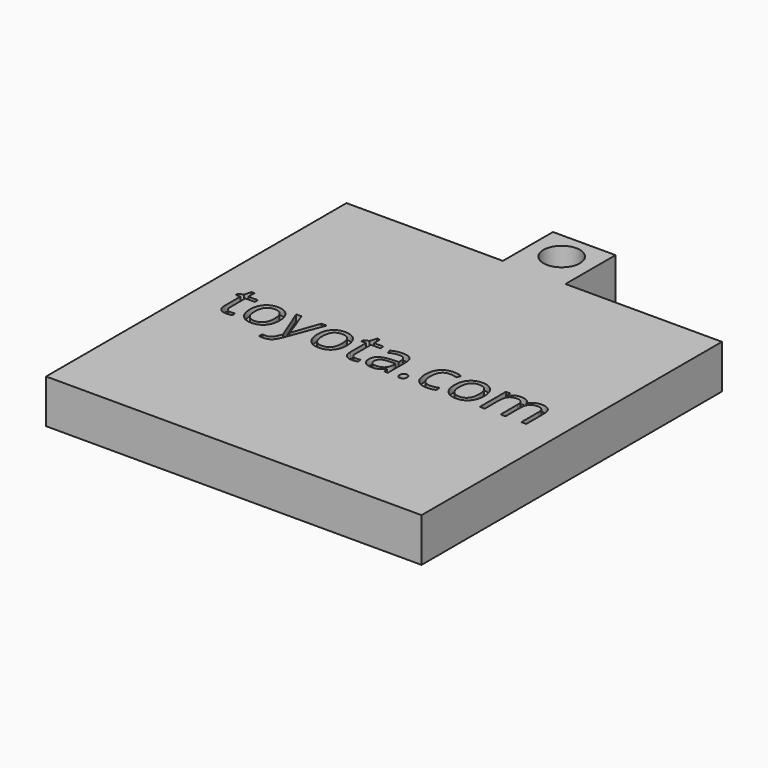
from build123d import *

# Parameters (mm, degrees)
F0_W          = 30
F0_H          = 30
F1_DEPTH      = 1.75
F2_W          = 5
F2_H          = 5
F3_DEPTH      = 3.5
F4_R          = 1.4562657213
F5_DEPTH      = 3.501
F7_DEPTH      = 0.5
F9_DEPTH      = 1.5
F11_DEPTH     = 1.5
F12_TEXT_SIZE = 4.8596224339
F13_DEPTH     = 0.5
F15_DEPTH     = 0.5
F16_W         = 3
F16_H         = 3
F16_W_2       = 2
F16_H_2       = 1
F17_DEPTH     = 0.5


# Not quite as in the source:
# - Text() gives the source's letters only with a copy of the font that has no kerning and outlines rounded to 1/6400 em; it was checked with that copy


with BuildPart() as f1:
    # F0 (on Top) → F1 (new body, symmetric)
    with BuildSketch(Plane.XY):
        Rectangle(F0_W, F0_H)
    extrude(amount=F1_DEPTH, both=True)

    # F2 (on face) → F3 (join)
    with BuildSketch(Plane.XY.offset(1.75)):
        with Locations((0, 17.5)):
            Rectangle(F2_W, F2_H)
    extrude(amount=-F3_DEPTH)

    # F4 (on face) → F5 (cut, through all)
    with BuildSketch(Plane.XY.offset(1.75)):
        with Locations((0, 17.7479702979)):
            Circle(F4_R)
    extrude(amount=-F5_DEPTH, mode=Mode.SUBTRACT)

    # F6 (on face) → F7 (cut)
    with BuildSketch(Plane(origin=(0, 0, -1.75), x_dir=(1, 0, 0), z_dir=(0, 0, -1))):
        Polygon((6.8512228218, 6), (-7.0022408961, 6), (-10, 3.3517099187), (-10, -3.3207885759), (-7.0298440874, -6), (7.0254140546, -6), (10, -3.3257078594), (10, 3.5331797223), align=None)
    extrude(amount=-F7_DEPTH, mode=Mode.SUBTRACT)

    # F8 (on face) → F9 (join)
    with BuildSketch(Plane(origin=(0, 0, -1.25), x_dir=(1, 0, 0), z_dir=(0, 0, -1))):
        Polygon((-7.5, 0), (-4.0358983849, -2), (4.1385644502, -2), (7.5, 0.1681215474), (7.5, 2), (4.1385644502, 1), (-4.0358983849, 1), (-7.5, 2), align=None)
    extrude(amount=F9_DEPTH)

    # F10 (on face) → F11 (join)
    with BuildSketch(Plane(origin=(0, 0, -1.25), x_dir=(1, 0, 0), z_dir=(0, 0, -1))):
        Polygon((-3, 2.6259386598), (-1.318838467, 1.5425661939), (1.3849237273, 1.5425661939), (3, 2.722196913), (3, 5.0425661939), (1.3849237273, 4.0425661939), (-1.318838467, 4.0425661939), (-3, 5.0425661939), align=None)
    extrude(amount=F11_DEPTH)

    # F12 (on face) → F13 (cut)
    with BuildSketch(Plane.XY.offset(1.75)):
        with Locations((-12.7181634307, -1.2958818082)):
            Text('toyota.com', F12_TEXT_SIZE, font='Open Sans', text_align=(TextAlign.LEFT, TextAlign.BOTTOM))
    extrude(amount=-F13_DEPTH, mode=Mode.SUBTRACT)

    # F14 (on face) → F15 (cut)
    with BuildSketch(Plane(origin=(0, 0, -1.75), x_dir=(1, 0, 0), z_dir=(0, 0, -1))):
        Polygon((11.3382770084, -10.5932966216), (10.1514638675, -10.5932966216), (10.1514638675, -8.0548351981), (9.5250901492, -8.0548351981), (9.5250901492, -10.6262634707), (8.3382770084, -10.6262634707), (8.3382770084, -11.0218674526), (11.3382770084, -11.0218674526), align=None)
    extrude(amount=-F15_DEPTH, mode=Mode.SUBTRACT)

    # F16 (on face) → F17 (cut)
    with BuildSketch(Plane(origin=(0, 0, -1.75), x_dir=(1, 0, 0), z_dir=(0, 0, -1))):
        with Locations((6.3382770084, -9.5218674526)):
            Rectangle(F16_W, F16_H)
        with Locations((6.3225585572, -9.5218674526)):
            Rectangle(F16_W_2, F16_H_2, mode=Mode.SUBTRACT)
    extrude(amount=-F17_DEPTH, mode=Mode.SUBTRACT)


solid = f1.part
